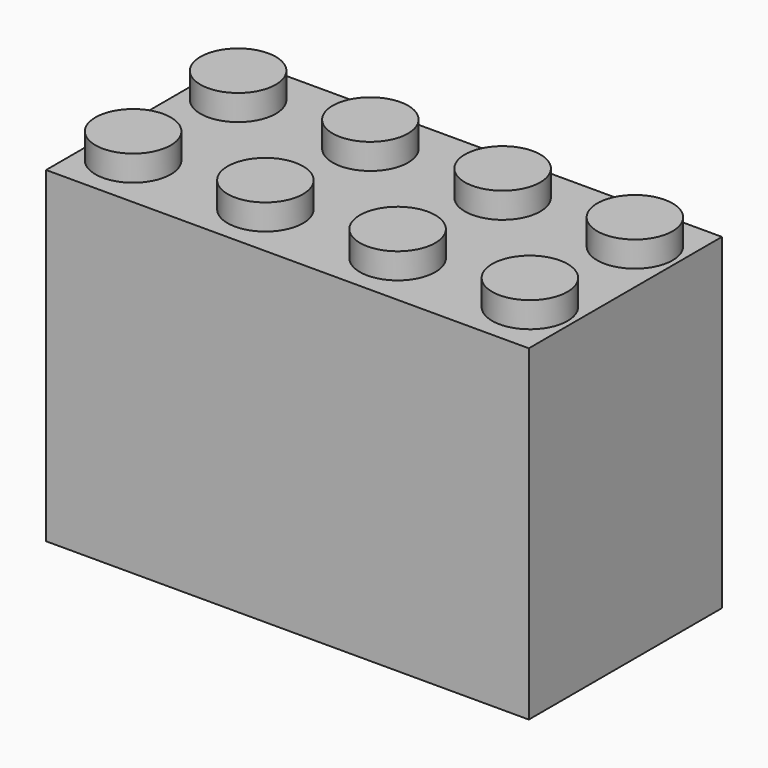
from build123d import *

# Parameters (mm, degrees)
F0_W     = 96
F0_H     = 48
F1_DEPTH = 65
F2_R     = 7.5
F3_DEPTH = 5.1
F4_T     = -2
F5_R     = 3.75
F5_R_2   = 3.25
F6_DEPTH = 63
F8_DEPTH = 6.5


# Not quite as in the source:
# - after a boolean that leaves OpenCascade's solid faulty, fix() repairs it


with BuildPart() as f1:
    # F0 (on Top) → F1 (new body)
    with BuildSketch(Plane.XY):
        Rectangle(F0_W, F0_H)
    extrude(amount=F1_DEPTH)

    # F2 (on face) → F3 (join)
    with BuildSketch(Plane.XY.offset(65)):
        with Locations((-39.45, 13.05)):
            Circle(F2_R)
        with Locations((-13.15, 13.05)):
            Circle(F2_R)
        with Locations((39.45, 13.05)):
            Circle(F2_R)
        with Locations((39.45, -13.05)):
            Circle(F2_R)
        with Locations((13.15, -13.05)):
            Circle(F2_R)
        with Locations((-13.15, -13.05)):
            Circle(F2_R)
        with Locations((-39.45, -13.05)):
            Circle(F2_R)
        with Locations((13.15, 13.05)):
            Circle(F2_R)
    extrude(amount=F3_DEPTH)

    # F4
    f4_openings = [f1.faces().sort_by_distance(p)[0] for p in [
        (0, 0, 0),
    ]]
    offset(amount=F4_T, openings=f4_openings, kind=Kind.INTERSECTION)

    # F5 (on face) → F6 (join, through all)
    with BuildSketch(Plane(origin=(0, 0, 63), x_dir=(1, 0, 0), z_dir=(0, 0, -1))):
        with Locations((-26.3, 0)):
            Circle(F5_R)
        with Locations((-26.3, 0)):
            Circle(F5_R_2, mode=Mode.SUBTRACT)
        with Locations((-18.1, 0)):
            Circle(F5_R)
        with Locations((-18.1, 0)):
            Circle(F5_R_2, mode=Mode.SUBTRACT)
        with Locations((-9.9, 0)):
            Circle(F5_R)
        with Locations((-9.9, 0)):
            Circle(F5_R_2, mode=Mode.SUBTRACT)
    extrude(amount=F6_DEPTH)

    # F7 (on face) → F8 (join)
    with BuildSketch(Plane(origin=(0, 0, 63), x_dir=(1, 0, 0), z_dir=(0, 0, -1))):
        with BuildLine():
            ThreePointArc((-20.1, 3.1721443851), (-18.1, 3.75), (-16.1, 3.1721443851))
            Line((-16.1, 3.1721443851), (-16.1, 8.4080715214))
            ThreePointArc((-16.1, 8.4080715214), (-18.65, 13.05), (-16.1, 17.6919284786))
            Line((-16.1, 17.6919284786), (-16.1, 22))
            Line((-16.1, 22), (-20.1, 22))
            Line((-20.1, 22), (-20.1, 3.1721443851))
        make_face()
        with BuildLine():
            Line((-16.1, -8.4080715214), (-16.1, -3.1721443851))
            ThreePointArc((-16.1, -3.1721443851), (-18.1, -3.75), (-20.1, -3.1721443851))
            Line((-20.1, -3.1721443851), (-20.1, -22))
            Line((-20.1, -22), (-16.1, -22))
            Line((-16.1, -22), (-16.1, -17.6919284786))
            ThreePointArc((-16.1, -17.6919284786), (-18.65, -13.05), (-16.1, -8.4080715214))
        make_face()
    extrude(amount=F8_DEPTH)

    add(f1.part.fix(), mode=Mode.REPLACE)


solid = f1.part
